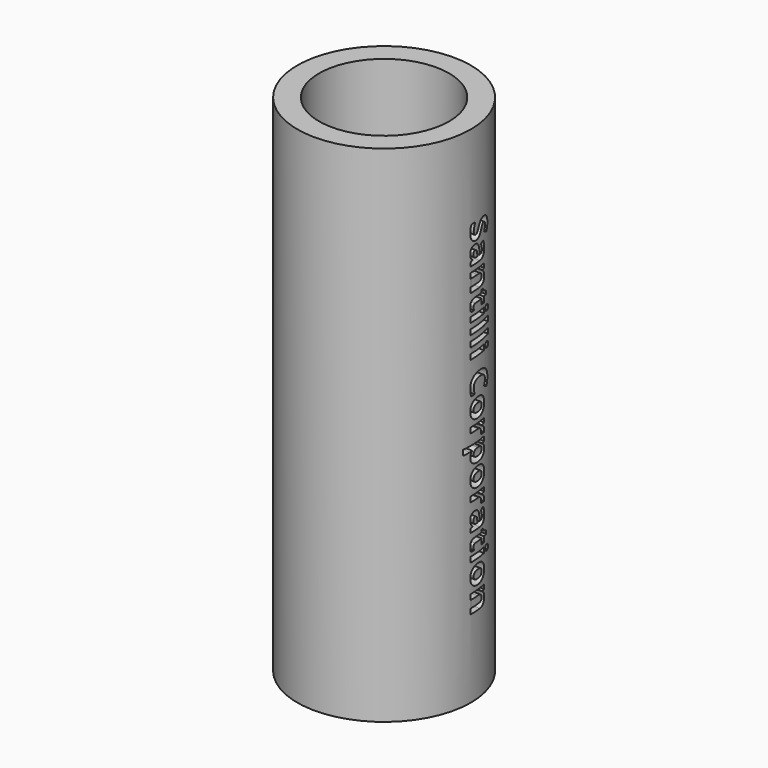
from build123d import *

# Parameters (mm, degrees)
F0_R         = 10
F0_R_2       = 7.5
F1_DEPTH     = 58.2
F3_TEXT_SIZE = 4.1015124327
F4_DEPTH     = 11.9


# Not quite as in the source:
# - Text() gives the source's letters only with a copy of the font that has no kerning and outlines rounded to 1/6400 em; it was checked with that copy


with BuildPart() as f1:
    # F0 (on Top) → F1 (new body)
    with BuildSketch(Plane.XY):
        Circle(F0_R)
        Circle(F0_R_2, mode=Mode.SUBTRACT)
    extrude(amount=F1_DEPTH)

    # F3 (on offset) → F4 (cut)
    with BuildSketch(Plane.YZ.offset(20)):
        with Locations(Location((-0.0398136438, 48.7000015378), (0, 0, -90))):
            Text('Santilli Corporation', F3_TEXT_SIZE, font='Open Sans', font_style=FontStyle.BOLD, text_align=(TextAlign.LEFT, TextAlign.BOTTOM))
    extrude(amount=-F4_DEPTH, mode=Mode.SUBTRACT)


solid = f1.part
